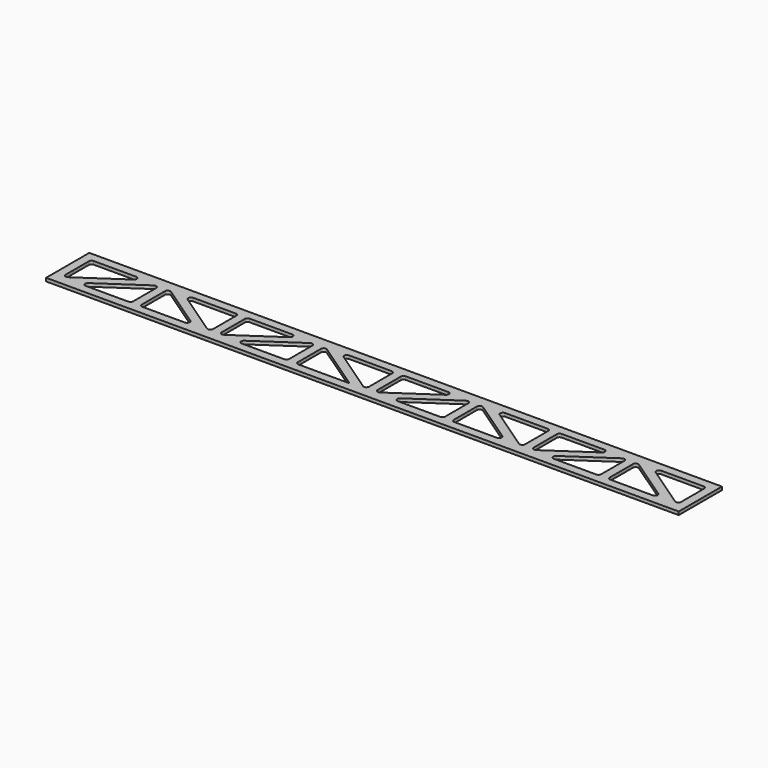
from build123d import *

# Parameters (mm, degrees)
F0_W     = 76.2270272544
F0_H     = 50
F1_DEPTH = 3


# Not quite as in the source:
# - a feature names something its author has since deleted; it is built from what else it names


with BuildPart() as f1:
    # F0 (on Top) → F1 (new body)
    with BuildSketch(Plane.XY):
        with Locations((38.1135136272, -25)):
            Rectangle(F0_W, F0_H)
        Polygon((8, -10.5), (8, -8), (10.5, -8), (49.8775833948, -8), (58, -8), (51.2833586059, -12.567316148), (11.9057752805, -39.3440728093), (8, -42), (8, -37.2767567084), align=None, mode=Mode.SUBTRACT)
        Polygon((68.3212522165, -10.6559270258), (72.2270272544, -8), (72.2270272544, -12.7232432916), (72.2270272544, -39.5), (72.2270272544, -42), (69.7270272544, -42), (30.3494438597, -42), (22.2270272544, -42), (28.9436687283, -37.4326837978), align=None, mode=Mode.SUBTRACT)
        Polygon((144.4540545089, 0), (76.2270272544, 0), (76.2270272544, -50), (144.4540545089, -50), (144.4540545089, -42), (140.5482796221, -39.344073077), (101.1706960016, -12.567316215), (94.4540545089, -8), (102.5764711141, -8), (141.9540545089, -8), (144.4540545089, -8), align=None)
        Polygon((80.2270272544, -8), (84.1328023313, -10.6559270523), (123.5103856735, -37.432683725), (130.2270272544, -42), (122.1046106492, -42), (82.7270272544, -42), (80.2270272544, -42), (80.2270272544, -39.5), (80.2270272544, -12.7232432967), align=None, mode=Mode.SUBTRACT)
        Polygon((152.4540545089, 0), (144.4540545089, 0), (144.4540545089, -8), (144.4540545089, -10.5), (144.4540545089, -37.2767567084), (144.4540545089, -42), (144.4540545089, -50), (152.4540545089, -50), (152.4540545089, -42), (152.4540545089, -37.2767567084), (152.4540545089, -10.5000000175), (152.4540545089, -8), align=None)
        Polygon((220.6810817633, 0), (152.4540545089, 0), (152.4540545089, -8), (154.9540545089, -8), (194.3316379036, -8), (202.4540545089, -8), (195.7374131063, -12.5673161537), (156.3598295468, -39.3440729742), (152.4540545089, -42), (152.4540545089, -50), (220.6810817633, -50), align=None)
        Polygon((212.7753064808, -10.6559271921), (216.6810817633, -8), (216.6810817633, -12.7232432916), (216.6810817633, -39.5), (216.6810817633, -42), (214.1810817633, -42), (174.8034983685, -42), (166.6810817633, -42), (173.3977233306, -37.4326837343), align=None, mode=Mode.SUBTRACT)
        with BuildLine():
            Line((144.4540545089, -10.5), (144.4540545089, -8))
            Line((144.4540545089, -8), (141.9540545089, -8))
            ThreePointArc((141.9540545089, -8), (143.7218214618, -8.732233047), (144.4540545089, -10.5))
        make_face()
        with BuildLine():
            Line((140.5482796221, -39.344073077), (144.4540545089, -42))
            Line((144.4540545089, -42), (144.4540545089, -37.2767567084))
            ThreePointArc((144.4540545089, -37.2767567084), (143.1235763734, -39.4863310132), (140.5482796221, -39.344073077))
        make_face()
        with BuildLine():
            Line((154.9540545089, -8), (152.4540545089, -8))
            Line((152.4540545089, -8), (152.4540545089, -10.5000000175))
            ThreePointArc((152.4540545089, -10.5000000175), (153.1862875497, -8.7322330532), (154.9540545089, -8))
        make_face()
        Polygon((288.9081090177, 0), (220.6810817633, 0), (220.6810817633, -50), (288.9081090177, -50), (288.9081090177, -42), (285.0023339882, -39.3440729799), (245.6247502909, -12.5673160658), (238.9081090177, -8), (247.030525623, -8), (286.4081090177, -8), (288.9081090177, -8), align=None)
        Polygon((224.6810817633, -8), (228.5868569969, -10.6559271589), (267.964440196, -37.4326837343), (274.6810817633, -42), (266.558665158, -42), (227.1810817633, -42), (224.6810817633, -42), (224.6810817633, -39.5), (224.6810817633, -12.7232432916), align=None, mode=Mode.SUBTRACT)
        with BuildLine():
            Line((152.4540545089, -37.2767567084), (152.4540545089, -42))
            Line((152.4540545089, -42), (156.3598295468, -39.3440729742))
            ThreePointArc((156.3598295468, -39.3440729742), (153.7845327252, -39.486331056), (152.4540545089, -37.2767567084))
        make_face()
        Polygon((296.9081090177, 0), (288.9081090177, 0), (288.9081090177, -8), (288.9081090177, -10.5), (288.9081090177, -37.2767567084), (288.9081090177, -42), (288.9081090177, -50), (296.9081090177, -50), (296.9081090177, -42), (296.9081090177, -37.2767567084), (296.9081090177, -10.4999999368), (296.9081090177, -8), align=None)
        with BuildLine():
            ThreePointArc((101.1706960016, -12.567316215), (100.1870893387, -9.7645717362), (102.5764711141, -8))
            Line((102.5764711141, -8), (94.4540545089, -8))
            Line((94.4540545089, -8), (101.1706960016, -12.567316215))
        make_face()
        with BuildLine():
            Line((202.4540545089, -8), (194.3316379036, -8))
            ThreePointArc((194.3316379036, -8), (196.0994048566, -8.732233047), (196.8316379036, -10.5))
            ThreePointArc((196.8316379036, -10.5), (196.5412122978, -11.6695216957), (195.7374131063, -12.5673161537))
            Line((195.7374131063, -12.5673161537), (202.4540545089, -8))
        make_face()
        Polygon((365.1351362721, 0), (296.9081090177, 0), (296.9081090177, -8), (299.4081090177, -8), (338.7856924125, -8), (346.9081090177, -8), (340.1914674861, -12.5673162415), (300.8138840557, -39.3440729742), (296.9081090177, -42), (296.9081090177, -50), (365.1351362721, -50), align=None)
        Polygon((357.2293616111, -10.6559267695), (361.1351362721, -8), (361.1351362721, -12.7232432916), (361.1351362721, -39.5), (361.1351362721, -42), (358.6351362721, -42), (319.2575528774, -42), (311.1351362721, -42), (317.8517779905, -37.4326836315), align=None, mode=Mode.SUBTRACT)
        with BuildLine():
            Line((288.9081090177, -10.5), (288.9081090177, -8))
            Line((288.9081090177, -8), (286.4081090177, -8))
            ThreePointArc((286.4081090177, -8), (288.1758759707, -8.732233047), (288.9081090177, -10.5))
        make_face()
        with BuildLine():
            Line((285.0023339882, -39.3440729799), (288.9081090177, -42))
            Line((288.9081090177, -42), (288.9081090177, -37.2767567084))
            ThreePointArc((288.9081090177, -37.2767567084), (287.5776308059, -39.4863310536), (285.0023339882, -39.3440729799))
        make_face()
        with BuildLine():
            Line((299.4081090177, -8), (296.9081090177, -8))
            Line((296.9081090177, -8), (296.9081090177, -10.4999999368))
            ThreePointArc((296.9081090177, -10.4999999368), (297.6403420871, -8.7322330247), (299.4081090177, -8))
        make_face()
        Polygon((433.3621635266, 0), (365.1351362721, 0), (365.1351362721, -50), (433.3621635266, -50), (433.3621635266, -42), (429.4563884885, -39.3440729741), (390.0788050582, -12.5673162415), (383.3621635266, -8), (391.4845801318, -8), (430.8621635266, -8), (433.3621635266, -8), align=None)
        Polygon((369.1351362721, -8), (373.0409110624, -10.6559268574), (412.4184949494, -37.4326839005), (419.1351362721, -42), (411.0127196669, -42), (371.6351362721, -42), (369.1351362721, -42), (369.1351362721, -39.5), (369.1351362721, -12.7232431652), align=None, mode=Mode.SUBTRACT)
        with BuildLine():
            Line((296.9081090177, -37.2767567084), (296.9081090177, -42))
            Line((296.9081090177, -42), (300.8138840557, -39.3440729742))
            ThreePointArc((300.8138840557, -39.3440729742), (298.238587234, -39.486331056), (296.9081090177, -37.2767567084))
        make_face()
        Polygon((441.3621635266, 0), (433.3621635266, 0), (433.3621635266, -8), (433.3621635266, -10.5), (433.3621635266, -37.2767567084), (433.3621635266, -42), (433.3621635266, -50), (441.3621635266, -50), (441.3621635266, -42), (441.3621635266, -37.2767567084), (441.3621635266, -10.4999999368), (441.3621635266, -8), align=None)
        with BuildLine():
            ThreePointArc((245.6247502909, -12.5673160658), (244.6411438866, -9.7645716093), (247.030525623, -8))
            Line((247.030525623, -8), (238.9081090177, -8))
            Line((238.9081090177, -8), (245.6247502909, -12.5673160658))
        make_face()
        with BuildLine():
            Line((346.9081090177, -8), (338.7856924125, -8))
            ThreePointArc((338.7856924125, -8), (340.5534593654, -8.732233047), (341.2856924125, -10.5))
            ThreePointArc((341.2856924125, -10.5), (340.9952667701, -11.6695217646), (340.1914674861, -12.5673162415))
            Line((340.1914674861, -12.5673162415), (346.9081090177, -8))
        make_face()
        Polygon((509.589190781, 0), (441.3621635266, 0), (441.3621635266, -8), (443.8621635266, -8), (483.2397469213, -8), (491.3621635266, -8), (484.6455219371, -12.5673162808), (445.2679384166, -39.3440730748), (441.3621635266, -42), (441.3621635266, -50), (509.589190781, -50), align=None)
        Polygon((501.6834161743, -10.6559267325), (505.589190781, -8), (505.589190781, -12.7232432916), (505.589190781, -39.5), (505.589190781, -42), (503.089190781, -42), (463.7116073862, -42), (455.589190781, -42), (462.3058321038, -37.4326839005), align=None, mode=Mode.SUBTRACT)
        with BuildLine():
            Line((433.3621635266, -10.5), (433.3621635266, -8))
            Line((433.3621635266, -8), (430.8621635266, -8))
            ThreePointArc((430.8621635266, -8), (432.6299304795, -8.732233047), (433.3621635266, -10.5))
        make_face()
        with BuildLine():
            Line((429.4563884885, -39.3440729741), (433.3621635266, -42))
            Line((433.3621635266, -42), (433.3621635266, -37.2767567084))
            ThreePointArc((433.3621635266, -37.2767567084), (432.0316853102, -39.486331056), (429.4563884885, -39.3440729741))
        make_face()
        with BuildLine():
            Line((443.8621635266, -8), (441.3621635266, -8))
            Line((441.3621635266, -8), (441.3621635266, -10.4999999368))
            ThreePointArc((441.3621635266, -10.4999999368), (442.0943965959, -8.7322330247), (443.8621635266, -8))
        make_face()
        with Locations((547.7027044082, -25)):
            Rectangle(F0_W, F0_H)
        Polygon((513.589190781, -8), (517.4949653468, -10.6559267047), (556.8725494042, -37.4326838638), (563.589190781, -42), (555.4667741758, -42), (516.089190781, -42), (513.589190781, -42), (513.589190781, -39.5), (513.589190781, -12.723243235), align=None, mode=Mode.SUBTRACT)
        Polygon((577.8162180354, -8), (577.8162180354, -10.5), (577.8162180354, -37.2767567084), (577.8162180354, -42), (573.9104428468, -39.3440728717), (534.5328596602, -12.5673163048), (527.8162180354, -8), (535.9386346407, -8), (575.3162180354, -8), align=None, mode=Mode.SUBTRACT)
        with BuildLine():
            Line((441.3621635266, -37.2767567084), (441.3621635266, -42))
            Line((441.3621635266, -42), (445.2679384166, -39.3440730748))
            ThreePointArc((445.2679384166, -39.3440730748), (442.6926416638, -39.4863310142), (441.3621635266, -37.2767567084))
        make_face()
        with BuildLine():
            ThreePointArc((390.0788050582, -12.5673162415), (389.0951983495, -9.7645717587), (391.4845801318, -8))
            Line((391.4845801318, -8), (383.3621635266, -8))
            Line((383.3621635266, -8), (390.0788050582, -12.5673162415))
        make_face()
        with BuildLine():
            Line((491.3621635266, -8), (483.2397469213, -8))
            ThreePointArc((483.2397469213, -8), (485.0075138743, -8.732233047), (485.7397469213, -10.5))
            ThreePointArc((485.7397469213, -10.5), (485.4493212626, -11.6695217955), (484.6455219371, -12.5673162808))
            Line((484.6455219371, -12.5673162808), (491.3621635266, -8))
        make_face()
        with BuildLine():
            Line((10.5, -8), (8, -8))
            Line((8, -8), (8, -10.5))
            ThreePointArc((8, -10.5), (8.732233047, -8.732233047), (10.5, -8))
        make_face()
        with BuildLine():
            Line((58, -8), (49.8775833948, -8))
            ThreePointArc((49.8775833948, -8), (51.6453503477, -8.732233047), (52.3775833948, -10.5))
            ThreePointArc((52.3775833948, -10.5), (52.0871577913, -11.6695216912), (51.2833586059, -12.567316148))
            Line((51.2833586059, -12.567316148), (58, -8))
        make_face()
        with BuildLine():
            ThreePointArc((11.9057752805, -39.3440728093), (9.3304783459, -39.4863311246), (8, -37.2767567084))
            Line((8, -37.2767567084), (8, -42))
            Line((8, -42), (11.9057752805, -39.3440728093))
        make_face()
        with BuildLine():
            Line((72.2270272544, -12.7232432916), (72.2270272544, -8))
            Line((72.2270272544, -8), (68.3212522165, -10.6559270258))
            ThreePointArc((68.3212522165, -10.6559270258), (70.8965490381, -10.513668944), (72.2270272544, -12.7232432916))
        make_face()
        with BuildLine():
            ThreePointArc((30.3494438597, -42), (27.9600620876, -40.2354282747), (28.9436687283, -37.4326837978))
            Line((28.9436687283, -37.4326837978), (22.2270272544, -42))
            Line((22.2270272544, -42), (30.3494438597, -42))
        make_face()
        with BuildLine():
            Line((72.2270272544, -42), (72.2270272544, -39.5))
            ThreePointArc((72.2270272544, -39.5), (71.4947942074, -41.267766953), (69.7270272544, -42))
            Line((69.7270272544, -42), (72.2270272544, -42))
        make_face()
        with BuildLine():
            ThreePointArc((80.2270272544, -12.7232432967), (81.5575054893, -10.5136689342), (84.1328023313, -10.6559270523))
            Line((84.1328023313, -10.6559270523), (80.2270272544, -8))
            Line((80.2270272544, -8), (80.2270272544, -12.7232432967))
        make_face()
        with BuildLine():
            Line((130.2270272544, -42), (123.5103856735, -37.432683725))
            ThreePointArc((123.5103856735, -37.432683725), (124.3141849929, -38.330478209), (124.6046106492, -39.5))
            ThreePointArc((124.6046106492, -39.5), (123.8723776022, -41.267766953), (122.1046106492, -42))
            Line((122.1046106492, -42), (130.2270272544, -42))
        make_face()
        with BuildLine():
            ThreePointArc((82.7270272544, -42), (80.9592603015, -41.267766953), (80.2270272544, -39.5))
            Line((80.2270272544, -39.5), (80.2270272544, -42))
            Line((80.2270272544, -42), (82.7270272544, -42))
        make_face()
        with BuildLine():
            Line((216.6810817633, -12.7232432916), (216.6810817633, -8))
            Line((216.6810817633, -8), (212.7753064808, -10.6559271921))
            ThreePointArc((212.7753064808, -10.6559271921), (215.3506034163, -10.5136688748), (216.6810817633, -12.7232432916))
        make_face()
        with BuildLine():
            ThreePointArc((174.8034983685, -42), (172.4141165798, -40.2354282207), (173.3977233306, -37.4326837343))
            Line((173.3977233306, -37.4326837343), (166.6810817633, -42))
            Line((166.6810817633, -42), (174.8034983685, -42))
        make_face()
        with BuildLine():
            Line((216.6810817633, -42), (216.6810817633, -39.5))
            ThreePointArc((216.6810817633, -39.5), (215.9488487163, -41.267766953), (214.1810817633, -42))
            Line((214.1810817633, -42), (216.6810817633, -42))
        make_face()
        with BuildLine():
            ThreePointArc((224.6810817633, -12.7232432916), (226.0115600842, -10.5136688886), (228.5868569969, -10.6559271589))
            Line((228.5868569969, -10.6559271589), (224.6810817633, -8))
            Line((224.6810817633, -8), (224.6810817633, -12.7232432916))
        make_face()
        with BuildLine():
            ThreePointArc((227.1810817633, -42), (225.4133148103, -41.267766953), (224.6810817633, -39.5))
            Line((224.6810817633, -39.5), (224.6810817633, -42))
            Line((224.6810817633, -42), (227.1810817633, -42))
        make_face()
        with BuildLine():
            Line((361.1351362721, -12.7232432916), (361.1351362721, -8))
            Line((361.1351362721, -8), (357.2293616111, -10.6559267695))
            ThreePointArc((357.2293616111, -10.6559267695), (359.8046582573, -10.5136690506), (361.1351362721, -12.7232432916))
        make_face()
        with BuildLine():
            ThreePointArc((319.2575528774, -42), (316.8681710618, -40.2354281334), (317.8517779905, -37.4326836315))
            Line((317.8517779905, -37.4326836315), (311.1351362721, -42))
            Line((311.1351362721, -42), (319.2575528774, -42))
        make_face()
        with BuildLine():
            Line((361.1351362721, -42), (361.1351362721, -39.5))
            ThreePointArc((361.1351362721, -39.5), (360.4029032251, -41.267766953), (358.6351362721, -42))
            Line((358.6351362721, -42), (361.1351362721, -42))
        make_face()
        with BuildLine():
            ThreePointArc((369.1351362721, -12.7232431652), (370.4656144119, -10.5136689845), (373.0409110624, -10.6559268574))
            Line((373.0409110624, -10.6559268574), (369.1351362721, -8))
            Line((369.1351362721, -8), (369.1351362721, -12.7232431652))
        make_face()
        with BuildLine():
            Line((419.1351362721, -42), (412.4184949494, -37.4326839005))
            ThreePointArc((412.4184949494, -37.4326839005), (413.2222940836, -38.330478347), (413.5127196669, -39.5))
            ThreePointArc((413.5127196669, -39.5), (412.7804866199, -41.267766953), (411.0127196669, -42))
            Line((411.0127196669, -42), (419.1351362721, -42))
        make_face()
        with BuildLine():
            ThreePointArc((371.6351362721, -42), (369.8673693192, -41.267766953), (369.1351362721, -39.5))
            Line((369.1351362721, -39.5), (369.1351362721, -42))
            Line((369.1351362721, -42), (371.6351362721, -42))
        make_face()
        with BuildLine():
            Line((505.589190781, -12.7232432916), (505.589190781, -8))
            Line((505.589190781, -8), (501.6834161743, -10.6559267325))
            ThreePointArc((501.6834161743, -10.6559267325), (504.2587127952, -10.513669066), (505.589190781, -12.7232432916))
        make_face()
        with BuildLine():
            ThreePointArc((463.7116073862, -42), (461.322225641, -40.235428362), (462.3058321038, -37.4326839005))
            Line((462.3058321038, -37.4326839005), (455.589190781, -42))
            Line((455.589190781, -42), (463.7116073862, -42))
        make_face()
        with BuildLine():
            Line((505.589190781, -42), (505.589190781, -39.5))
            ThreePointArc((505.589190781, -39.5), (504.856957734, -41.267766953), (503.089190781, -42))
            Line((503.089190781, -42), (505.589190781, -42))
        make_face()
        with BuildLine():
            ThreePointArc((575.3162180354, -8), (577.0839849884, -8.732233047), (577.8162180354, -10.5))
            Line((577.8162180354, -10.5), (577.8162180354, -8))
            Line((577.8162180354, -8), (575.3162180354, -8))
        make_face()
        with BuildLine():
            Line((577.8162180354, -42), (577.8162180354, -37.2767567084))
            ThreePointArc((577.8162180354, -37.2767567084), (576.4857397386, -39.4863310986), (573.9104428468, -39.3440728717))
            Line((573.9104428468, -39.3440728717), (577.8162180354, -42))
        make_face()
        with BuildLine():
            ThreePointArc((534.5328596602, -12.5673163048), (533.5492528418, -9.7645718125), (535.9386346407, -8))
            Line((535.9386346407, -8), (527.8162180354, -8))
            Line((527.8162180354, -8), (534.5328596602, -12.5673163048))
        make_face()
        with BuildLine():
            ThreePointArc((513.589190781, -12.723243235), (514.91966877, -10.5136690643), (517.4949653468, -10.6559267047))
            Line((517.4949653468, -10.6559267047), (513.589190781, -8))
            Line((513.589190781, -8), (513.589190781, -12.723243235))
        make_face()
        with BuildLine():
            Line((563.589190781, -42), (556.8725494042, -37.4326838638))
            ThreePointArc((556.8725494042, -37.4326838638), (557.6763485772, -38.3304783181), (557.9667741758, -39.5))
            ThreePointArc((557.9667741758, -39.5), (557.2345411287, -41.267766953), (555.4667741758, -42))
            Line((555.4667741758, -42), (563.589190781, -42))
        make_face()
        with BuildLine():
            ThreePointArc((516.089190781, -42), (514.321423828, -41.267766953), (513.589190781, -39.5))
            Line((513.589190781, -39.5), (513.589190781, -42))
            Line((513.589190781, -42), (516.089190781, -42))
        make_face()
    extrude(amount=F1_DEPTH)


solid = f1.part
